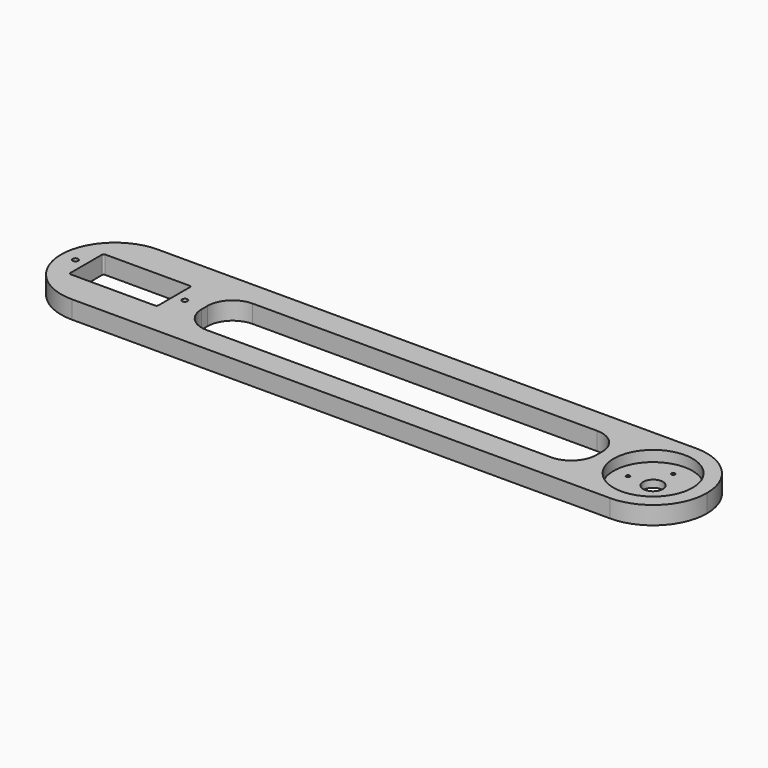
from build123d import *

# Parameters (mm, degrees)
F0_W     = 180
F0_H     = 30
F0_W_2   = 110
F0_H_2   = 16
F1_DEPTH = 5
F2_R     = 11
F2_R_2   = 0.5
F2_R_3   = 2.75
F2_W     = 24.5
F2_H     = 12
F3_DEPTH = 3
F2_R_4   = 0.75
F4_DEPTH = 25
F5_R     = 14.99999
F6_R     = 7
F7_R     = 0.5


# Not quite as in the source:
# - a fillet or chamfer is up to 0.001 mm smaller than in the source, because OpenCascade refuses the exact size
# - a feature names something its author has since deleted; it is built from what else it names


with BuildPart() as f1:
    # F0 (on Top) → F1 (new body)
    with BuildSketch(Plane.XY):
        with Locations((10, -11.8972941886)):
            Rectangle(F0_W, F0_H)
        with Locations((15, -11.8972941886)):
            Rectangle(F0_W_2, F0_H_2, mode=Mode.SUBTRACT)
    extrude(amount=F1_DEPTH)

    # F2 (on face) → F3 (cut)
    with BuildSketch(Plane.XY.offset(5)):
        with Locations((85, -11.8972941886)):
            Circle(F2_R)
        with Locations((85, -18.8972941886)):
            Circle(F2_R_2, mode=Mode.SUBTRACT)
        with Locations((85, -11.8972941886)):
            Circle(F2_R_3, mode=Mode.SUBTRACT)
        with Locations((78, -11.8972941886)):
            Circle(F2_R_2, mode=Mode.SUBTRACT)
        with Locations((92, -11.8972941886)):
            Circle(F2_R_2, mode=Mode.SUBTRACT)
        with Locations((85, -4.8972941886)):
            Circle(F2_R_2, mode=Mode.SUBTRACT)
        with Locations((-60.75, -11.8972941886)):
            Rectangle(F2_W, F2_H)
        with Locations((-65, -11.8972941886)):
            Circle(F2_R_3, mode=Mode.SUBTRACT)
    extrude(amount=-F3_DEPTH, mode=Mode.SUBTRACT)

    # F2 (on face) → F4 (cut)
    with BuildSketch(Plane.XY.offset(5)):
        with Locations((-60.75, -11.8972941886)):
            Rectangle(F2_W, F2_H)
        with Locations((-65, -11.8972941886)):
            Circle(F2_R_3, mode=Mode.SUBTRACT)
        with Locations((85, -11.8972941886)):
            Circle(F2_R_3)
        with Locations((-65, -11.8972941886)):
            Circle(F2_R_3)
        with Locations((-76, -11.8972941886)):
            Circle(F2_R_4)
        with Locations((-45.5, -11.8972941886)):
            Circle(F2_R_4)
        with Locations((85, -4.8972941886)):
            Circle(F2_R_2)
        with Locations((78, -11.8972941886)):
            Circle(F2_R_2)
        with Locations((85, -18.8972941886)):
            Circle(F2_R_2)
        with Locations((92, -11.8972941886)):
            Circle(F2_R_2)
    extrude(amount=-F4_DEPTH, mode=Mode.SUBTRACT)

    # F5 (radius 15 in the source; OpenCascade refuses exactly that, so slightly less here)
    f5_edges = [f1.edges().sort_by_distance(p)[0] for p in [
        (100, 3.102706, 2.5),
        (100, -26.897294, 2.5),
        (-80, -26.897294, 2.5),
        (-80, 3.102706, 2.5),
    ]]
    fillet(f5_edges, radius=F5_R)

    # F6
    f6_edges = [f1.edges().sort_by_distance(p)[0] for p in [
        (-40, -3.897294, 2.5),
        (-40, -19.897294, 2.5),
        (70, -3.897294, 2.5),
        (70, -19.897294, 2.5),
    ]]
    fillet(f6_edges, radius=F6_R)

    # F7
    f7_edges = [f1.edges().sort_by_distance(p)[0] for p in [
        (-73, -5.897294, 2.5),
        (-73, -17.897294, 2.5),
        (-48.5, -5.897294, 2.5),
        (-48.5, -17.897294, 2.5),
    ]]
    fillet(f7_edges, radius=F7_R)


solid = f1.part
